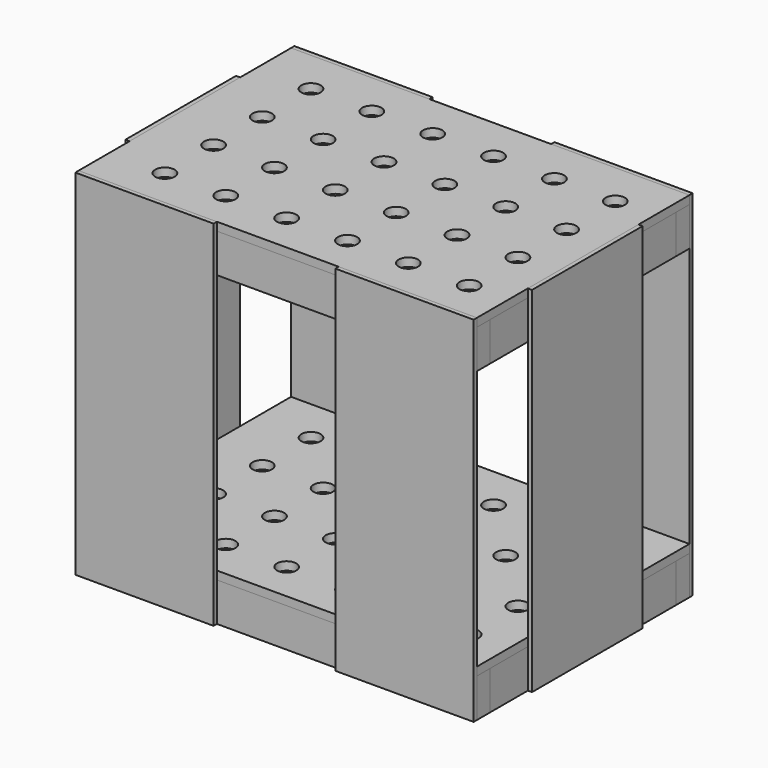
from build123d import *

# Parameters (mm, degrees)
F0_W      = 914.4
F0_H      = 88.9
F1_DEPTH  = 38.1
F2_W      = 38.1
F2_H      = 88.9
F3_DEPTH  = 533.4
F6_W      = 914.4
F6_H      = 609.6
F7_DEPTH  = 19.05
F8_R      = 22.225
F9_DEPTH  = 19.05
F10_W     = 317.5
F10_H     = 812.8
F11_DEPTH = 9.525
F15_ANGLE = -90


with BuildPart() as f1:
    # F0 (on Front) → F1 (new body)
    with BuildSketch(Plane.XZ):
        with Locations((457.2, -44.45)):
            Rectangle(F0_W, F0_H)
    extrude(amount=F1_DEPTH)


with BuildPart() as f3:
    # F2 (on face) → F3 (new body)
    with BuildSketch(Plane(origin=(0, 0, 0), x_dir=(-1, 0, 0), z_dir=(0, 1, 0))):
        with Locations((-895.35, -44.45)):
            Rectangle(F2_W, F2_H)
    extrude(amount=F3_DEPTH)


with BuildPart() as f4_1:
    # F4: copy of F3
    add(f3.part.moved(Location((-876.3, 0, 0))))


with BuildPart() as f5_1:
    # F5: copy of F1
    add(f1.part.moved(Location((0, 571.5, 0))))


with BuildPart() as f7:
    # F6 (on Top) → F7 (new body)
    with BuildSketch(Plane.XY):
        with Locations((457.2, 266.7)):
            Rectangle(F6_W, F6_H)
    extrude(amount=F7_DEPTH)

    # F8 (on Top) → F9 (cut, through all)
    with BuildSketch(Plane.XY):
        with Locations((266.7, 330.2)):
            Circle(F8_R)
        with Locations((546.1, 190.5)):
            Circle(F8_R)
        with Locations((127, 190.5)):
            Circle(F8_R)
        with Locations((825.5, 190.5)):
            Circle(F8_R)
        with Locations((825.5, 50.8)):
            Circle(F8_R)
        with Locations((406.4, 330.2)):
            Circle(F8_R)
        with Locations((406.4, 190.5)):
            Circle(F8_R)
        with Locations((406.4, 469.9)):
            Circle(F8_R)
        with Locations((127, 50.8)):
            Circle(F8_R)
        with Locations((406.4, 50.8)):
            Circle(F8_R)
        with Locations((546.1, 330.2)):
            Circle(F8_R)
        with Locations((546.1, 469.9)):
            Circle(F8_R)
        with Locations((266.7, 50.8)):
            Circle(F8_R)
        with Locations((127, 330.2)):
            Circle(F8_R)
        with Locations((546.1, 50.8)):
            Circle(F8_R)
        with Locations((685.8, 469.9)):
            Circle(F8_R)
        with Locations((825.5, 469.9)):
            Circle(F8_R)
        with Locations((825.5, 330.2)):
            Circle(F8_R)
        with Locations((266.7, 190.5)):
            Circle(F8_R)
        with Locations((127, 469.9)):
            Circle(F8_R)
        with Locations((685.8, 330.2)):
            Circle(F8_R)
        with Locations((266.7, 469.9)):
            Circle(F8_R)
        with Locations((685.8, 190.5)):
            Circle(F8_R)
        with Locations((685.8, 50.8)):
            Circle(F8_R)
    extrude(amount=F9_DEPTH, mode=Mode.SUBTRACT)


with BuildPart() as f11:
    # F10 (on Right) → F11 (new body)
    with BuildSketch(Plane.YZ):
        with Locations((120.65, 317.5)):
            Rectangle(F10_W, F10_H)
    extrude(amount=-F11_DEPTH)


with BuildPart() as f12_1:
    # F12: copy of F11
    add(f11.part.moved(Location((923.925, 0, 0))))


with BuildPart() as f13_1:
    # F13: copy of F1
    add(f1.part.moved(Location((0, 0, 704.85))))


with BuildPart() as f13_2:
    # F13: copy of F3
    add(f3.part.moved(Location((0, 0, 704.85))))


with BuildPart() as f13_3:
    # F13: copy of F4_1
    add(f4_1.part.moved(Location((0, 0, 704.85))))


with BuildPart() as f13_4:
    # F13: copy of F5_1
    add(f5_1.part.moved(Location((0, 0, 704.85))))


with BuildPart() as f13_5:
    # F13: copy of F7
    add(f7.part.moved(Location((0, 0, 704.85))))


with BuildPart() as f14_1:
    # F14: copy of F11
    add(f11.part.moved(Location((0, 609.6, 0))))


with BuildPart() as f14_1_1:
    # F15: moved
    add(f14_1.part.rotate(Axis((0, 571.5, 317.5), (0, 0, 1)), F15_ANGLE))


with BuildPart() as f16_1:
    # F16: copy of F14_1
    add(f14_1_1.part.moved(Location((596.9, 0, 0))))


with BuildPart() as f17_1:
    # F17: copy of F16_1
    add(f16_1.part.moved(Location((0, -619.125, 0))))


with BuildPart() as f18_1:
    # F18: copy of F14_1
    add(f14_1_1.part.moved(Location((0, -619.125, 0))))


with BuildPart() as f11_1:
    # F19: moved
    add(f11.part.moved(Location((0, 146.05, 0))))


with BuildPart() as f12_1_1:
    # F20: moved
    add(f12_1.part.moved(Location((0, 146.05, 0))))


solid = Compound([f1.part, f3.part, f4_1.part, f5_1.part, f7.part, f13_1.part, f13_2.part, f13_3.part, f13_4.part, f13_5.part, f14_1_1.part, f16_1.part, f17_1.part, f18_1.part, f11_1.part, f12_1_1.part])
